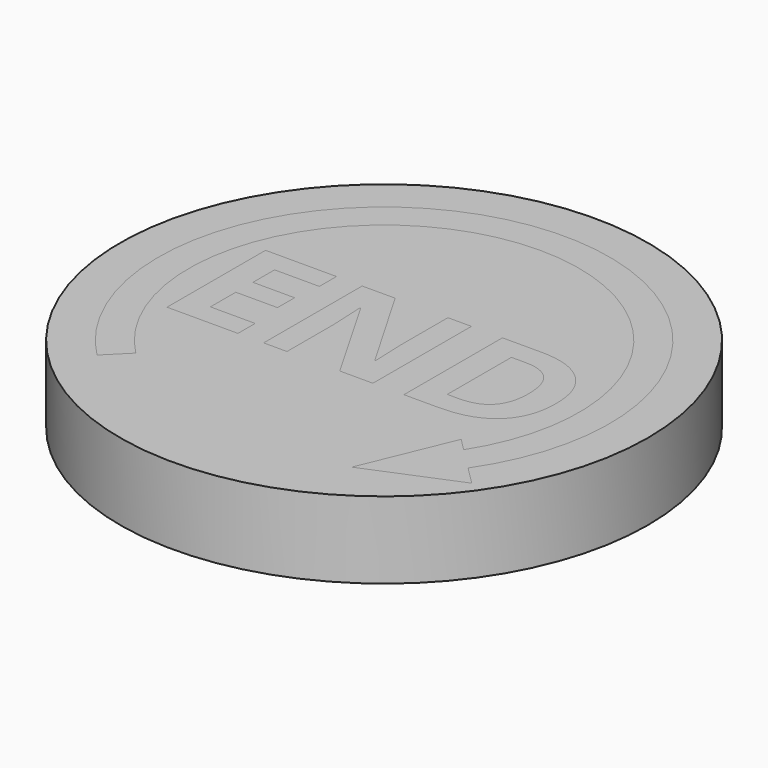
from build123d import *

# Parameters (mm, degrees)
F0_R         = 21.65
F1_DEPTH     = 6.3
F3_DEPTH     = 1
F4_TEXT_SIZE = 14.1509433962
F5_DEPTH     = 0.5
F7_DEPTH     = 1
F8_DEPTH     = 0.5


# Not quite as in the source:
# - Text() gives the source's letters only with a copy of the font that has no kerning and outlines rounded to 1/6400 em; it was checked with that copy


with BuildPart() as f1:
    # F0 (on Top) → F1 (new body)
    with BuildSketch(Plane.XY):
        Circle(F0_R)
    extrude(amount=F1_DEPTH)

    # F2 (on face) → F3 (cut)
    with BuildSketch(Plane.XY.offset(6.3)):
        with BuildLine():
            ThreePointArc((-11.313708499, -11.313708499), (-1.7052303324, 15.9088714092), (13.4545166696, -8.6588672001))
            Line((13.4545166696, -8.6588672001), (12.4306323096, -7.6349828401))
            Line((12.4306323096, -7.6349828401), (9.3691648507, -15.0260191002))
            Line((9.3691648507, -15.0260191002), (16.7602011108, -11.9645516413))
            Line((16.7602011108, -11.9645516413), (15.2576628574, -10.4620133879))
            ThreePointArc((15.2576628574, -10.4620133879), (-1.7027458067, 18.4214727076), (-13.081475452, -13.081475452))
            Line((-13.081475452, -13.081475452), (-11.313708499, -11.313708499))
        make_face()
    extrude(amount=-F3_DEPTH, mode=Mode.SUBTRACT)

    # F4 (on face) → F5 (cut)
    with BuildSketch(Plane.XY.offset(6.3)):
        with Locations((-15, -5.0943396226)):
            Text('END', F4_TEXT_SIZE, font='Open Sans', font_style=FontStyle.BOLD, text_align=(TextAlign.LEFT, TextAlign.BOTTOM))
    extrude(amount=-F5_DEPTH, mode=Mode.SUBTRACT)


with BuildPart() as f7:
    # F6 (on face) → F7 (new body, through all)
    with BuildSketch(Plane.XY.offset(6.3)):
        with BuildLine():
            Line((-13.081475452, -13.081475452), (-11.313708499, -11.313708499))
            ThreePointArc((-11.313708499, -11.313708499), (-1.7052303324, 15.9088714092), (13.4545166696, -8.6588672001))
            Line((13.4545166696, -8.6588672001), (12.4306323096, -7.6349828401))
            Line((12.4306323096, -7.6349828401), (9.3691648507, -15.0260191002))
            Line((9.3691648507, -15.0260191002), (16.7602011108, -11.9645516413))
            Line((16.7602011108, -11.9645516413), (15.2576628574, -10.4620133879))
            ThreePointArc((15.2576628574, -10.4620133879), (-1.7027458067, 18.4214727076), (-13.081475452, -13.081475452))
        make_face()
    extrude(amount=-F7_DEPTH)


with BuildPart() as f8:
    # F4 (on face) → F8 (new body, through all)
    with BuildSketch(Plane.XY.offset(6.3)):
        with Locations((-15, -5.0943396226)):
            Text('END', F4_TEXT_SIZE, font='Open Sans', font_style=FontStyle.BOLD, text_align=(TextAlign.LEFT, TextAlign.BOTTOM))
    extrude(amount=-F8_DEPTH)


solid = Compound([f1.part, f7.part, f8.part])
